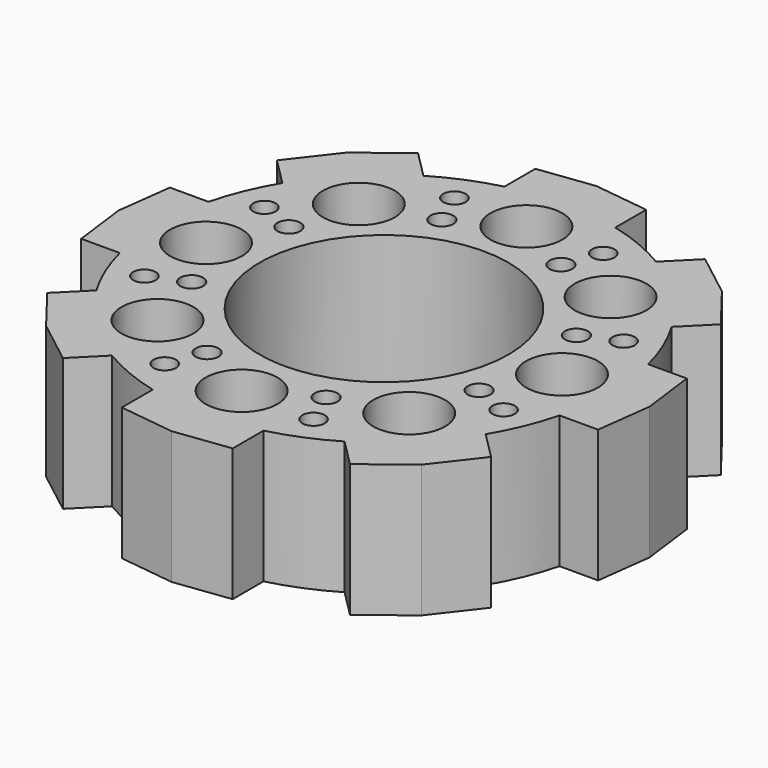
from build123d import *

# Parameters (mm, degrees)
F1_R     = 2.1084229829
F1_R_2   = 2.1529922124
F1_R_3   = 6.765859494
F1_R_4   = 23.4458713357
F2_DEPTH = 12.5


# Not quite as in the source:
# - ends of sketch curves that miss each other by under 0.0002 mm in the source are joined


with BuildPart() as f2:
    # F1 (on Top) → F2 (new body, symmetric)
    with BuildSketch(Plane.XY):
        with BuildLine():
            Line((10.4387272149, 48.6714951694), (-2.1118e-06, 50))
            Line((-2.1118e-06, 50), (-10.4387272149, 48.6714951694))
            Line((-10.4387272149, 48.6714951694), (-10.4387272149, 41.4038337767))
            ThreePointArc((-10.4387272149, 41.4038337767), (-16.3403785702, 39.4491635584), (-21.89563683, 36.6582264313))
            Line((-21.89563683, 36.6582264313), (-27.0346494841, 41.7972390854))
            Line((-27.0346494841, 41.7972390854), (-35.3553405526, 35.355337566))
            Line((-35.3553405526, 35.355337566), (-41.7972390854, 27.0346494841))
            Line((-41.7972390854, 27.0346494841), (-36.6582264313, 21.89563683))
            ThreePointArc((-36.6582264313, 21.89563683), (-39.4491635584, 16.3403785702), (-41.4038337767, 10.4387272149))
            Line((-41.4038337767, 10.4387272149), (-48.6714951694, 10.4387272149))
            Line((-48.6714951694, 10.4387272149), (-50, -2.1118e-06))
            Line((-50, -2.1118e-06), (-48.6714951694, -10.4387272149))
            Line((-48.6714951694, -10.4387272149), (-41.4038337767, -10.4387272149))
            ThreePointArc((-41.4038337767, -10.4387272149), (-39.4491635584, -16.3403785702), (-36.6582264313, -21.89563683))
            Line((-36.6582264313, -21.89563683), (-41.7972390854, -27.0346494841))
            Line((-41.7972390854, -27.0346494841), (-35.355337566, -35.3553405526))
            Line((-35.355337566, -35.3553405526), (-27.0346494841, -41.7972390854))
            Line((-27.0346494841, -41.7972390854), (-21.89563683, -36.6582264313))
            ThreePointArc((-21.89563683, -36.6582264313), (-16.3403785702, -39.4491635584), (-10.4387272149, -41.4038337767))
            Line((-10.4387272149, -41.4038337767), (-10.4387272149, -48.6714951694))
            Line((-10.4387272149, -48.6714951694), (2.1118e-06, -50))
            Line((2.1118e-06, -50), (10.4387272149, -48.6714951694))
            Line((10.4387272149, -48.6714951694), (10.4387272149, -41.4038337767))
            ThreePointArc((10.4387272149, -41.4038337767), (16.3403785702, -39.4491635584), (21.89563683, -36.6582264313))
            Line((21.89563683, -36.6582264313), (27.0346494841, -41.7972390854))
            Line((27.0346494841, -41.7972390854), (35.3553405526, -35.355337566))
            Line((35.3553405526, -35.355337566), (41.7972390854, -27.0346494841))
            Line((41.7972390854, -27.0346494841), (36.6582264313, -21.89563683))
            ThreePointArc((36.6582264313, -21.89563683), (39.4491635584, -16.3403785702), (41.4038337767, -10.4387272149))
            Line((41.4038337767, -10.4387272149), (48.6714951694, -10.4387272149))
            Line((48.6714951694, -10.4387272149), (50, 2.1118e-06))
            Line((50, 2.1118e-06), (48.6714951694, 10.4387272149))
            Line((48.6714951694, 10.4387272149), (41.4038337767, 10.4387272149))
            ThreePointArc((41.4038337767, 10.4387272149), (39.4491635584, 16.3403785702), (36.6582264313, 21.89563683))
            Line((36.6582264313, 21.89563683), (41.7972390854, 27.0346494841))
            Line((41.7972390854, 27.0346494841), (35.355337566, 35.3553405526))
            Line((35.355337566, 35.3553405526), (27.0346494841, 41.7972390854))
            Line((27.0346494841, 41.7972390854), (21.89563683, 36.6582264313))
            ThreePointArc((21.89563683, 36.6582264313), (16.3403785702, 39.4491635584), (10.4387272149, 41.4038337767))
            Line((10.4387272149, 41.4038337767), (10.4387272149, 48.6714951694))
        make_face()
        with Locations((-14.1885686223, -33.8735479302)):
            Circle(F1_R, mode=Mode.SUBTRACT)
        with Locations((-11.5808588113, -27.1737373769)):
            Circle(F1_R_2, mode=Mode.SUBTRACT)
        with Locations((-33.9850485325, -13.9193823561)):
            Circle(F1_R, mode=Mode.SUBTRACT)
        with Locations((-27.4036377668, -11.025830172)):
            Circle(F1_R_2, mode=Mode.SUBTRACT)
        with Locations((-23.7041544531, -23.7041544531)):
            Circle(F1_R_3, mode=Mode.SUBTRACT)
        with Locations((0, -33.5227367122)):
            Circle(F1_R_3, mode=Mode.SUBTRACT)
        with Locations((11.025830172, -27.4036377668)):
            Circle(F1_R_2, mode=Mode.SUBTRACT)
        with Locations((13.9193823561, -33.9850485325)):
            Circle(F1_R, mode=Mode.SUBTRACT)
        with Locations((23.7041544531, -23.7041544531)):
            Circle(F1_R_3, mode=Mode.SUBTRACT)
        with Locations((33.8735479302, -14.1885686223)):
            Circle(F1_R, mode=Mode.SUBTRACT)
        with Locations((27.1737373769, -11.5808588113)):
            Circle(F1_R_2, mode=Mode.SUBTRACT)
        with Locations((-33.5227367122, 0)):
            Circle(F1_R_3, mode=Mode.SUBTRACT)
        with Locations((-27.1737373769, 11.5808588113)):
            Circle(F1_R_2, mode=Mode.SUBTRACT)
        with Locations((-33.8735479302, 14.1885686223)):
            Circle(F1_R, mode=Mode.SUBTRACT)
        with Locations((-23.7041544531, 23.7041544531)):
            Circle(F1_R_3, mode=Mode.SUBTRACT)
        with Locations((-13.9193823561, 33.9850485325)):
            Circle(F1_R, mode=Mode.SUBTRACT)
        with Locations((-11.025830172, 27.4036377668)):
            Circle(F1_R_2, mode=Mode.SUBTRACT)
        Circle(F1_R_4, mode=Mode.SUBTRACT)
        with Locations((23.7041544531, 23.7041544531)):
            Circle(F1_R_3, mode=Mode.SUBTRACT)
        with Locations((33.5227367122, 0)):
            Circle(F1_R_3, mode=Mode.SUBTRACT)
        with Locations((27.4036377668, 11.025830172)):
            Circle(F1_R_2, mode=Mode.SUBTRACT)
        with Locations((33.9850485325, 13.9193823561)):
            Circle(F1_R, mode=Mode.SUBTRACT)
        with Locations((11.5808588113, 27.1737373769)):
            Circle(F1_R_2, mode=Mode.SUBTRACT)
        with Locations((0, 33.5227367122)):
            Circle(F1_R_3, mode=Mode.SUBTRACT)
        with Locations((14.1885686223, 33.8735479302)):
            Circle(F1_R, mode=Mode.SUBTRACT)
    extrude(amount=F2_DEPTH, both=True)


solid = f2.part
